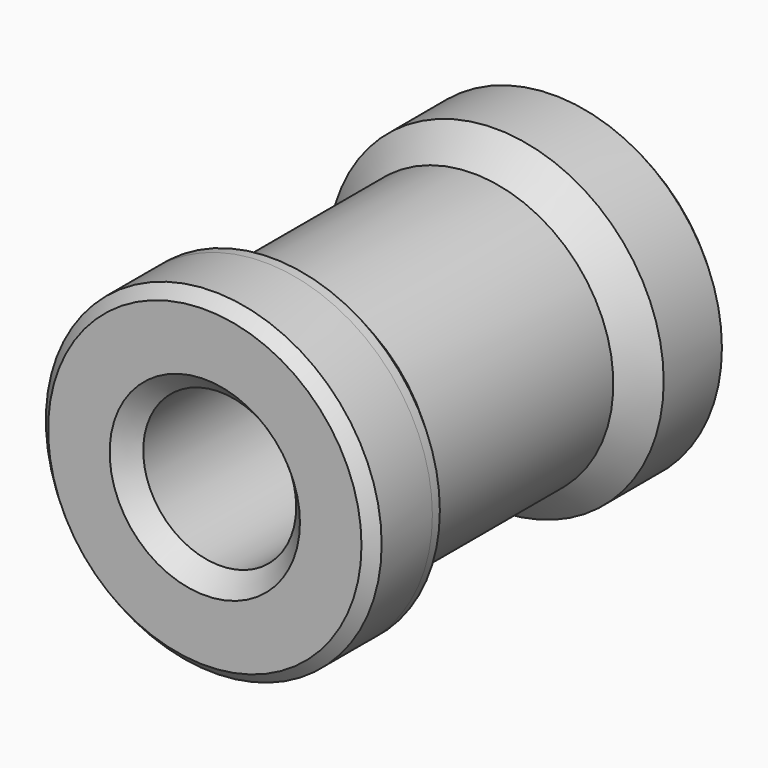
from build123d import *

# Parameters (mm, degrees)
F0_R         = 4.5
F0_R_2       = 2.05
F1_DEPTH     = 12
F2_SIZE      = 0.3
F3_SIZE      = 0.5
F4_SIZE      = 0.5
F5_SIZE      = 0.3
F6_W         = 0.7801173814
F6_H         = 8
F8_S5_R      = 4.5
F8_T6_DEPTH  = 8
F8_S11_R     = 4.5
F8_T12_DEPTH = 8


# Not quite as in the source:
# - a fillet or chamfer that OpenCascade refuses, or shapes differently, is made with other operations: its cross-section is extruded or revolved along the edge and cut away or added


with BuildPart() as f1:
    # F0 (on Front) → F1 (new body)
    with BuildSketch(Plane.XZ):
        Circle(F0_R)
        Circle(F0_R_2, mode=Mode.SUBTRACT)
    extrude(amount=F1_DEPTH)

    # F2
    f2_edges = [f1.edges().sort_by_distance(p)[0] for p in [
        (-4.5, -12, 0),
    ]]
    chamfer(f2_edges, length=F2_SIZE)

    # F3
    f3_edges = [f1.edges().sort_by_distance(p)[0] for p in [
        (-2.05, -12, 0),
    ]]
    chamfer(f3_edges, length=F3_SIZE)

    # F4
    f4_edges = [f1.edges().sort_by_distance(p)[0] for p in [
        (-2.05, 0, 0),
    ]]
    chamfer(f4_edges, length=F4_SIZE)

    # F5
    f5_edges = [f1.edges().sort_by_distance(p)[0] for p in [
        (-4.5, 0, 0),
    ]]
    chamfer(f5_edges, length=F5_SIZE)

    # F6 (on Top) → F7 (revolve, cut)
    with BuildSketch(Plane.XY):
        with Locations((-4.1400586907, -6)):
            Rectangle(F6_W, F6_H)
    revolve(axis=Axis((0, 2.6414038148, 0), (0, 1, 0)), mode=Mode.SUBTRACT)

    # F8: chamfer of 1 on 3 edges, made by hand


with BuildPart() as f8_tool2:
    # F8_s3 → F8_t4 (revolve)
    with BuildSketch(Plane.XY):
        Polygon((-3.75, -9), (-4.75, -10), (-3.75, -10), align=None)
    revolve(axis=Axis((0, -10, 0), (0, 1, 0)))

    # F8_s5 → F8_t6 (intersect, symmetric)
    with BuildSketch(Plane.XZ.offset(9.5)):
        Circle(F8_S5_R)
    extrude(amount=F8_T6_DEPTH, both=True, mode=Mode.INTERSECT)


with BuildPart() as f1_1:
    add(f1.part)

    # F8_t1: union F8_tool2
    add(f8_tool2.part)


with BuildPart() as f8_tool8:
    # F8_s9 → F8_t10 (revolve)
    with BuildSketch(Plane.XY):
        Polygon((-4.75, -2), (-3.75, -3), (-3.75, -2), align=None)
    revolve(axis=Axis((0, -2, 0), (0, 1, 0)))

    # F8_s11 → F8_t12 (intersect, symmetric)
    with BuildSketch(Plane.XZ.offset(2.5)):
        Circle(F8_S11_R)
    extrude(amount=F8_T12_DEPTH, both=True, mode=Mode.INTERSECT)


with BuildPart() as f1_2:
    add(f1_1.part)

    # F8_t7: union F8_tool8
    add(f8_tool8.part)


solid = f1_2.part
